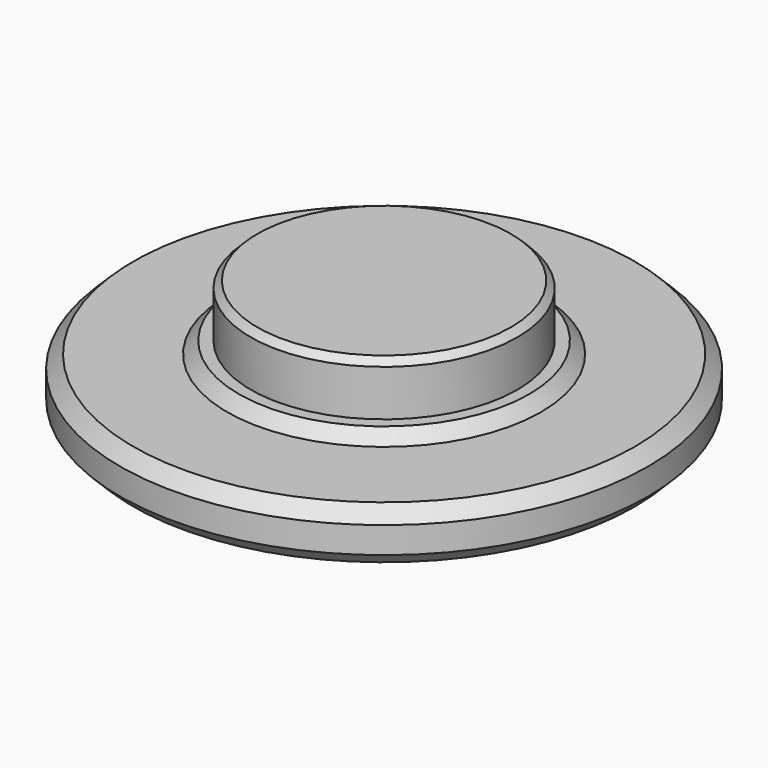
from build123d import *

# Parameters (mm, degrees)
F0_R     = 10
F1_DEPTH = 2
F2_R     = 6
F3_DEPTH = 0.45
F4_R     = 5.05
F5_DEPTH = 2
F6_SIZE  = 0.25
F8_SIZE  = 0.5


# Not quite as in the source:
# - a fillet or chamfer that OpenCascade refuses, or shapes differently, is made with other operations: its cross-section is extruded or revolved along the edge and cut away or added


with BuildPart() as f1:
    # F0 (on Top) → F1 (new body)
    with BuildSketch(Plane.XY):
        Circle(F0_R)
    extrude(amount=F1_DEPTH)

    # F2 (on face) → F3 (join)
    with BuildSketch(Plane.XY.offset(2)):
        Circle(F2_R)
    extrude(amount=F3_DEPTH)

    # F4 (on face) → F5 (join)
    with BuildSketch(Plane.XY.offset(2.45)):
        Circle(F4_R)
    extrude(amount=F5_DEPTH)

    # F6
    f6_edges = [f1.edges().sort_by_distance(p)[0] for p in [
        (-5.05, 0, 4.45),
    ]]
    chamfer(f6_edges, length=F6_SIZE)

    # F7: chamfer of 0.5 on 1 edges, made by hand


with BuildPart() as f7_tool2:
    # F7_s3 → F7_t4 (revolve)
    with BuildSketch(Plane.XZ):
        Polygon((5.5, 2.45), (6, 1.95), (6, 2.45), align=None)
    revolve(axis=Axis((0, 0, 2.45), (0, 0, 1)))

    split(bisect_by=Plane.XY.offset(2), keep=Keep.TOP)


with BuildPart() as f1_1:
    add(f1.part)

    # F7_t1: cut F7_tool2
    add(f7_tool2.part, mode=Mode.SUBTRACT)

    # F8
    f8_edges = [f1_1.edges().sort_by_distance(p)[0] for p in [
        (-10, 0, 0),
        (-10, 0, 2),
    ]]
    chamfer(f8_edges, length=F8_SIZE)


solid = f1_1.part
